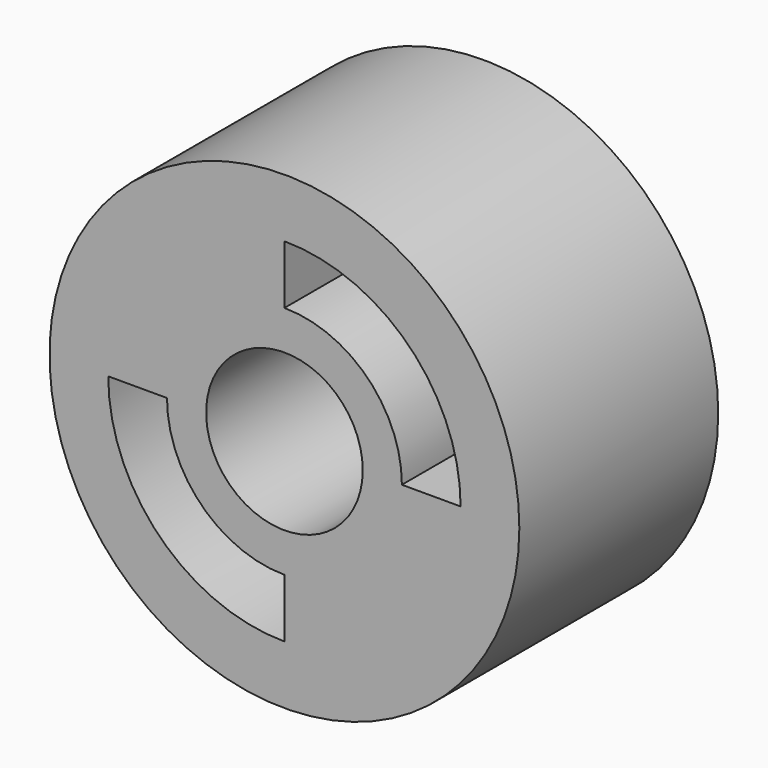
from build123d import *

# Parameters (mm, degrees)
F0_R     = 6
F0_R_2   = 2
F1_DEPTH = 6.35


# Not quite as in the source:
# - a length typed as a fraction of an inch, garbled in the dataset ("3 / 203.2 mm" for 3/8 in), is restored


with BuildPart() as f1:
    # F0 (on Front) → F1 (new body)
    with BuildSketch(Plane.XZ):
        Circle(F0_R)
        with BuildLine():
            ThreePointArc((0, 4.5), (3.1819805153, 3.1819805153), (4.5, 0))
            ThreePointArc((4.5, 0), (3.1819805153, -3.1819805153), (0, -4.5))
            ThreePointArc((0, -4.5), (-3.1819805153, -3.1819805153), (-4.5, 0))
            ThreePointArc((-4.5, 0), (-3.1819805153, 3.1819805153), (0, 4.5))
        make_face(mode=Mode.SUBTRACT)
        with BuildLine():
            ThreePointArc((0, -4.5), (3.1819805153, -3.1819805153), (4.5, 0))
            Line((4.5, 0), (3, 0))
            ThreePointArc((3, 0), (2.1213203436, -2.1213203436), (0, -3))
            Line((0, -3), (0, -4.5))
        make_face()
        with BuildLine():
            ThreePointArc((0, -3), (2.1213203436, -2.1213203436), (3, 0))
            ThreePointArc((3, 0), (2.1213203436, 2.1213203436), (0, 3))
            ThreePointArc((0, 3), (-2.1213203436, 2.1213203436), (-3, 0))
            ThreePointArc((-3, 0), (-2.1213203436, -2.1213203436), (0, -3))
        make_face()
        Circle(F0_R_2, mode=Mode.SUBTRACT)
        with BuildLine():
            Line((0, 3), (0, 4.5))
            ThreePointArc((0, 4.5), (-3.1819805153, 3.1819805153), (-4.5, 0))
            Line((-4.5, 0), (-3, 0))
            ThreePointArc((-3, 0), (-2.1213203436, 2.1213203436), (0, 3))
        make_face()
    extrude(amount=F1_DEPTH)


solid = f1.part
